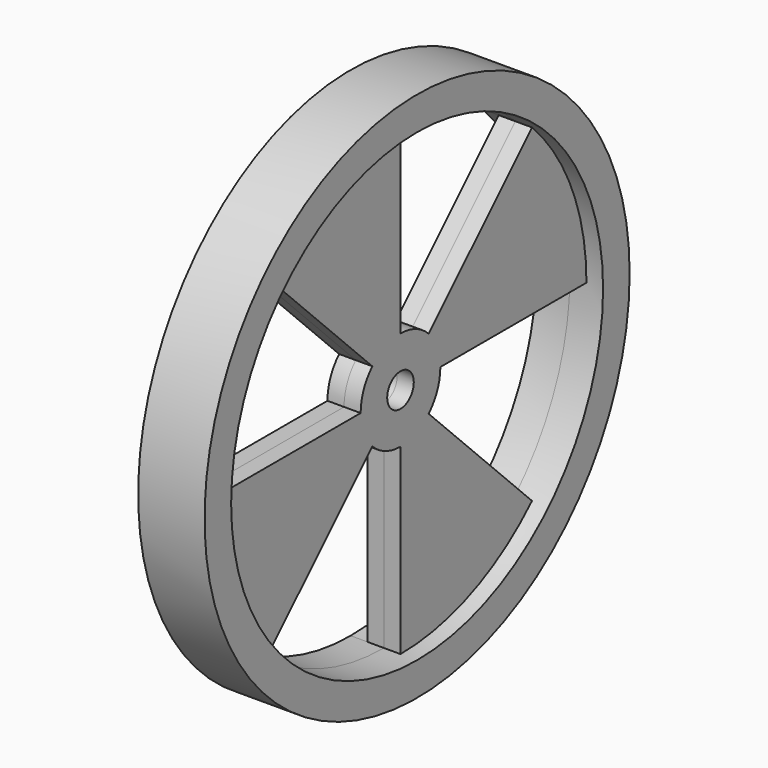
from build123d import *
from build123d import SkipClean  # not in build123d's __all__

# Parameters (mm, degrees)
F0_R       = 25.4
F1_DEPTH   = 6.35
F2_R       = 1.5875
F3_DEPTH   = 3.175
F4_DEPTH   = 1.5875
F5_R       = 1.5875
F3_FACE4_R = 1.5875
F4_FACE_R  = 1.5875
F6_DEPTH   = 1.5875
F7_DEPTH   = 3.175


with BuildPart() as f1:
    # F0 (on Right) → F1 (new body)
    with BuildSketch(Plane.YZ):
        Circle(F0_R)
    extrude(amount=F1_DEPTH)

    # F2 (on face) → F3 (cut)
    with BuildSketch(Plane.YZ.offset(6.35)):
        with BuildLine():
            Line((-3.3675960454, 3.3675960454), (-15.7154482119, 15.7154482119))
            ThreePointArc((-15.7154482119, 15.7154482119), (-20.5332226101, 8.5051392843), (-22.225, 0))
            Line((-22.225, 0), (-4.7625, 0))
            ThreePointArc((-4.7625, 0), (-4.3999762736, 1.8225298466), (-3.3675960454, 3.3675960454))
        make_face()
        with BuildLine():
            ThreePointArc((-15.7154482119, -15.7154482119), (-8.5051392843, -20.5332226101), (0, -22.225))
            Line((0, -22.225), (0, -4.7625))
            ThreePointArc((0, -4.7625), (-1.8225298466, -4.3999762736), (-3.3675960454, -3.3675960454))
            Line((-3.3675960454, -3.3675960454), (-15.7154482119, -15.7154482119))
        make_face()
        with BuildLine():
            ThreePointArc((15.7154482119, -15.7154482119), (20.5332226101, -8.5051392843), (22.225, 0))
            Line((22.225, 0), (4.7625, 0))
            ThreePointArc((4.7625, 0), (4.3999762736, -1.8225298466), (3.3675960454, -3.3675960454))
            Line((3.3675960454, -3.3675960454), (15.7154482119, -15.7154482119))
        make_face()
        with BuildLine():
            Line((3.3675960454, 3.3675960454), (15.7154482119, 15.7154482119))
            ThreePointArc((15.7154482119, 15.7154482119), (8.5051392843, 20.5332226101), (0, 22.225))
            Line((0, 22.225), (0, 4.7625))
            ThreePointArc((0, 4.7625), (1.8225298466, 4.3999762736), (3.3675960454, 3.3675960454))
        make_face()
        Circle(F2_R)
    extrude(amount=-F3_DEPTH, mode=Mode.SUBTRACT)

    # F2 (on face) → F4 (cut)
    with BuildSketch(Plane.YZ.offset(6.35)):
        with BuildLine():
            Line((0, 4.7625), (0, 22.225))
            ThreePointArc((0, 22.225), (-8.5051392843, 20.5332226101), (-15.7154482119, 15.7154482119))
            Line((-15.7154482119, 15.7154482119), (-3.3675960454, 3.3675960454))
            ThreePointArc((-3.3675960454, 3.3675960454), (-1.8225298466, 4.3999762736), (0, 4.7625))
        make_face()
        with BuildLine():
            Line((4.7625, 0), (22.225, 0))
            ThreePointArc((22.225, 0), (20.5332226101, 8.5051392843), (15.7154482119, 15.7154482119))
            Line((15.7154482119, 15.7154482119), (3.3675960454, 3.3675960454))
            ThreePointArc((3.3675960454, 3.3675960454), (4.3999762736, 1.8225298466), (4.7625, 0))
        make_face()
        with BuildLine():
            ThreePointArc((0, -22.225), (8.5051392843, -20.5332226101), (15.7154482119, -15.7154482119))
            Line((15.7154482119, -15.7154482119), (3.3675960454, -3.3675960454))
            ThreePointArc((3.3675960454, -3.3675960454), (1.8225298466, -4.3999762736), (0, -4.7625))
            Line((0, -4.7625), (0, -22.225))
        make_face()
        with BuildLine():
            ThreePointArc((-22.225, 0), (-20.5332226101, -8.5051392843), (-15.7154482119, -15.7154482119))
            Line((-15.7154482119, -15.7154482119), (-3.3675960454, -3.3675960454))
            ThreePointArc((-3.3675960454, -3.3675960454), (-4.3999762736, -1.8225298466), (-4.7625, 0))
            Line((-4.7625, 0), (-22.225, 0))
        make_face()
        with BuildLine():
            ThreePointArc((3.3675960454, -3.3675960454), (4.3999762736, -1.8225298466), (4.7625, 0))
            ThreePointArc((4.7625, 0), (4.3999762736, 1.8225298466), (3.3675960454, 3.3675960454))
            ThreePointArc((3.3675960454, 3.3675960454), (1.8225298466, 4.3999762736), (0, 4.7625))
            ThreePointArc((0, 4.7625), (-1.8225298466, 4.3999762736), (-3.3675960454, 3.3675960454))
            ThreePointArc((-3.3675960454, 3.3675960454), (-4.3999762736, 1.8225298466), (-4.7625, 0))
            ThreePointArc((-4.7625, 0), (-4.3999762736, -1.8225298466), (-3.3675960454, -3.3675960454))
            ThreePointArc((-3.3675960454, -3.3675960454), (-1.8225298466, -4.3999762736), (0, -4.7625))
            ThreePointArc((0, -4.7625), (1.8225298466, -4.3999762736), (3.3675960454, -3.3675960454))
        make_face()
        Circle(F2_R, mode=Mode.SUBTRACT)
    extrude(amount=-F4_DEPTH, mode=Mode.SUBTRACT)

    # F5 (on face) + F3_face (on face) + F3_face1 (on face) + F3_face2 (on face) + F3_face3 (on face) + F3_face4 (on face) + F4_face (on face) → F6 (cut)
    with BuildSketch(Plane(origin=(0, 0, 0), x_dir=(0, -1, 0), z_dir=(-1, 0, 0))):
        with BuildLine():
            Line((3.3675960454, 3.3675960454), (15.7154482119, 15.7154482119))
            ThreePointArc((15.7154482119, 15.7154482119), (8.5051392843, 20.5332226101), (0, 22.225))
            Line((0, 22.225), (0, 4.7625))
            ThreePointArc((0, 4.7625), (1.8225298466, 4.3999762736), (3.3675960454, 3.3675960454))
        make_face()
        with BuildLine():
            ThreePointArc((15.7154482119, -15.7154482119), (20.5332226101, -8.5051392843), (22.225, 0))
            Line((22.225, 0), (4.7625, 0))
            ThreePointArc((4.7625, 0), (4.3999762736, -1.8225298466), (3.3675960454, -3.3675960454))
            Line((3.3675960454, -3.3675960454), (15.7154482119, -15.7154482119))
        make_face()
        with BuildLine():
            ThreePointArc((-15.7154482119, -15.7154482119), (-8.5051392843, -20.5332226101), (0, -22.225))
            Line((0, -22.225), (0, -4.7625))
            ThreePointArc((0, -4.7625), (-1.8225298466, -4.3999762736), (-3.3675960454, -3.3675960454))
            Line((-3.3675960454, -3.3675960454), (-15.7154482119, -15.7154482119))
        make_face()
        with BuildLine():
            Line((-3.3675960454, 3.3675960454), (-15.7154482119, 15.7154482119))
            ThreePointArc((-15.7154482119, 15.7154482119), (-20.5332226101, 8.5051392843), (-22.225, 0))
            Line((-22.225, 0), (-4.7625, 0))
            ThreePointArc((-4.7625, 0), (-4.3999762736, 1.8225298466), (-3.3675960454, 3.3675960454))
        make_face()
        with BuildLine():
            ThreePointArc((3.3675960454, -3.3675960454), (4.3999762736, -1.8225298466), (4.7625, 0))
            ThreePointArc((4.7625, 0), (4.3999762736, 1.8225298466), (3.3675960454, 3.3675960454))
            ThreePointArc((3.3675960454, 3.3675960454), (1.8225298466, 4.3999762736), (0, 4.7625))
            ThreePointArc((0, 4.7625), (-1.8225298466, 4.3999762736), (-3.3675960454, 3.3675960454))
            ThreePointArc((-3.3675960454, 3.3675960454), (-4.3999762736, 1.8225298466), (-4.7625, 0))
            ThreePointArc((-4.7625, 0), (-4.3999762736, -1.8225298466), (-3.3675960454, -3.3675960454))
            ThreePointArc((-3.3675960454, -3.3675960454), (-1.8225298466, -4.3999762736), (0, -4.7625))
            ThreePointArc((0, -4.7625), (1.8225298466, -4.3999762736), (3.3675960454, -3.3675960454))
        make_face()
        Circle(F5_R, mode=Mode.SUBTRACT)
    with BuildSketch(Plane(origin=(3.175, -13.844128687, 5.7344258614), x_dir=(0, 1, 0), z_dir=(1, 0, 0))):
        with BuildLine():
            ThreePointArc((-1.8713195248, 9.9810223505), (-6.689093923, 2.7707134229), (-8.380871313, -5.7344258614))
            Line((-8.380871313, -5.7344258614), (9.081628687, -5.7344258614))
            ThreePointArc((9.081628687, -5.7344258614), (9.4441524134, -3.9118960148), (10.4765326416, -2.366829816))
            Line((10.4765326416, -2.366829816), (-1.8713195248, 9.9810223505))
        make_face()
    with BuildSketch(Plane(origin=(3.175, -5.7344258614, -13.844128687), x_dir=(0, 1, 0), z_dir=(1, 0, 0))):
        with BuildLine():
            ThreePointArc((-9.9810223505, -1.8713195248), (-2.7707134229, -6.689093923), (5.7344258614, -8.380871313))
            Line((5.7344258614, -8.380871313), (5.7344258614, 9.081628687))
            ThreePointArc((5.7344258614, 9.081628687), (3.9118960148, 9.4441524134), (2.366829816, 10.4765326416))
            Line((2.366829816, 10.4765326416), (-9.9810223505, -1.8713195248))
        make_face()
    with BuildSketch(Plane(origin=(3.175, 13.844128687, -5.7344258614), x_dir=(0, 1, 0), z_dir=(1, 0, 0))):
        with BuildLine():
            Line((-10.4765326416, 2.366829816), (1.8713195248, -9.9810223505))
            ThreePointArc((1.8713195248, -9.9810223505), (6.689093923, -2.7707134229), (8.380871313, 5.7344258614))
            Line((8.380871313, 5.7344258614), (-9.081628687, 5.7344258614))
            ThreePointArc((-9.081628687, 5.7344258614), (-9.4441524134, 3.9118960148), (-10.4765326416, 2.366829816))
        make_face()
    with BuildSketch(Plane(origin=(3.175, 5.7344258614, 13.844128687), x_dir=(0, 1, 0), z_dir=(1, 0, 0))):
        with BuildLine():
            ThreePointArc((9.9810223505, 1.8713195248), (2.7707134229, 6.689093923), (-5.7344258614, 8.380871313))
            Line((-5.7344258614, 8.380871313), (-5.7344258614, -9.081628687))
            ThreePointArc((-5.7344258614, -9.081628687), (-3.9118960148, -9.4441524134), (-2.366829816, -10.4765326416))
            Line((-2.366829816, -10.4765326416), (9.9810223505, 1.8713195248))
        make_face()
    with BuildSketch(Plane.YZ.offset(3.175)):
        Circle(F3_FACE4_R)
    with BuildSketch(Plane.YZ.offset(4.7625)):
        with BuildLine():
            Line((-15.7154482119, 15.7154482119), (-3.3675960454, 3.3675960454))
            ThreePointArc((-3.3675960454, 3.3675960454), (-4.3999762736, 1.8225298466), (-4.7625, 0))
            Line((-4.7625, 0), (-22.225, 0))
            ThreePointArc((-22.225, 0), (-20.5332226101, -8.5051392843), (-15.7154482119, -15.7154482119))
            Line((-15.7154482119, -15.7154482119), (-3.3675960454, -3.3675960454))
            ThreePointArc((-3.3675960454, -3.3675960454), (-1.8225298466, -4.3999762736), (0, -4.7625))
            Line((0, -4.7625), (0, -22.225))
            ThreePointArc((0, -22.225), (8.5051392843, -20.5332226101), (15.7154482119, -15.7154482119))
            Line((15.7154482119, -15.7154482119), (3.3675960454, -3.3675960454))
            ThreePointArc((3.3675960454, -3.3675960454), (4.3999762736, -1.8225298466), (4.7625, 0))
            Line((4.7625, 0), (22.225, 0))
            ThreePointArc((22.225, 0), (20.5332226101, 8.5051392843), (15.7154482119, 15.7154482119))
            Line((15.7154482119, 15.7154482119), (3.3675960454, 3.3675960454))
            ThreePointArc((3.3675960454, 3.3675960454), (1.8225298466, 4.3999762736), (0, 4.7625))
            Line((0, 4.7625), (0, 22.225))
            ThreePointArc((0, 22.225), (-8.5051392843, 20.5332226101), (-15.7154482119, 15.7154482119))
        make_face()
        Circle(F4_FACE_R, mode=Mode.SUBTRACT)
    extrude(amount=-F6_DEPTH, dir=(-1, 0, 0), mode=Mode.SUBTRACT)

    # F5 (on face) → F7 (cut)
    with BuildSketch(Plane(origin=(0, 0, 0), x_dir=(0, -1, 0), z_dir=(-1, 0, 0))):
        with BuildLine():
            Line((0, 4.7625), (0, 22.225))
            ThreePointArc((0, 22.225), (-8.5051392843, 20.5332226101), (-15.7154482119, 15.7154482119))
            Line((-15.7154482119, 15.7154482119), (-3.3675960454, 3.3675960454))
            ThreePointArc((-3.3675960454, 3.3675960454), (-1.8225298466, 4.3999762736), (0, 4.7625))
        make_face()
        with BuildLine():
            ThreePointArc((-22.225, 0), (-20.5332226101, -8.5051392843), (-15.7154482119, -15.7154482119))
            Line((-15.7154482119, -15.7154482119), (-3.3675960454, -3.3675960454))
            ThreePointArc((-3.3675960454, -3.3675960454), (-4.3999762736, -1.8225298466), (-4.7625, 0))
            Line((-4.7625, 0), (-22.225, 0))
        make_face()
        with BuildLine():
            ThreePointArc((0, -22.225), (8.5051392843, -20.5332226101), (15.7154482119, -15.7154482119))
            Line((15.7154482119, -15.7154482119), (3.3675960454, -3.3675960454))
            ThreePointArc((3.3675960454, -3.3675960454), (1.8225298466, -4.3999762736), (0, -4.7625))
            Line((0, -4.7625), (0, -22.225))
        make_face()
        with BuildLine():
            Line((4.7625, 0), (22.225, 0))
            ThreePointArc((22.225, 0), (20.5332226101, 8.5051392843), (15.7154482119, 15.7154482119))
            Line((15.7154482119, 15.7154482119), (3.3675960454, 3.3675960454))
            ThreePointArc((3.3675960454, 3.3675960454), (4.3999762736, 1.8225298466), (4.7625, 0))
        make_face()
        Circle(F5_R)
    with SkipClean():  # cleaning this boolean's faces spoils the solid; the shape is the same uncleaned
        extrude(amount=-F7_DEPTH, mode=Mode.SUBTRACT)


solid = f1.part
